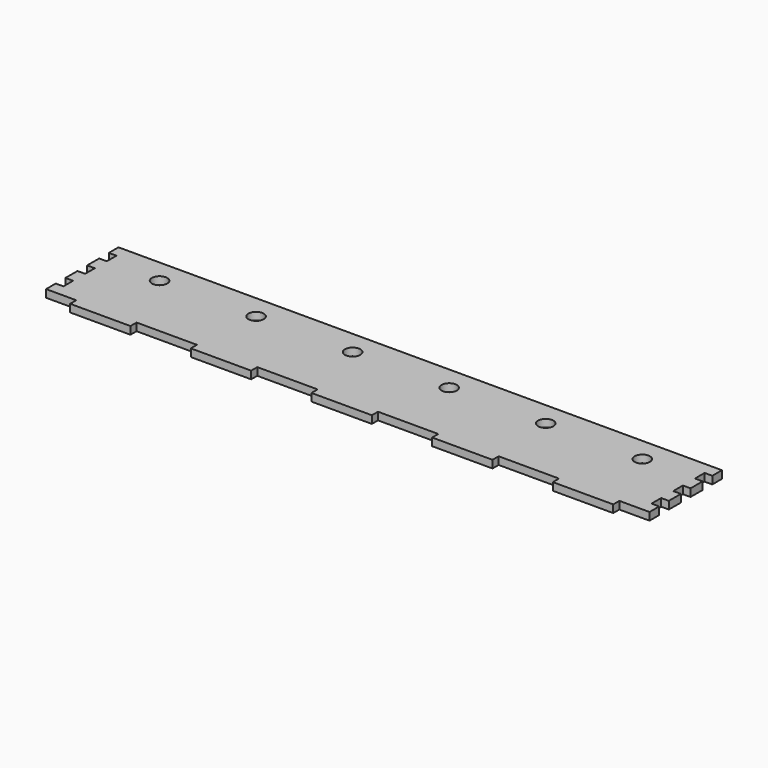
from build123d import *

# Parameters (mm, degrees)
F0_W     = 500
F0_H     = 75
F1_DEPTH = 6.35
F2_W     = 50
F2_H     = 6.35
F3_DEPTH = 6.35
F4_W     = 6.35
F4_H     = 10
F5_DEPTH = 6.351
F6_R     = 6.35
F7_DEPTH = 25


# Not quite as in the source:
# - a length typed as a fraction of an inch, garbled in the dataset ("3 / 203.2 mm" for 3/8 in), is restored


with BuildPart() as f1:
    # F0 (on Top) → F1 (new body)
    with BuildSketch(Plane.XY):
        Rectangle(F0_W, F0_H)
    extrude(amount=F1_DEPTH)

    # F2 (on face) → F3 (join, through all)
    with BuildSketch(Plane.XY.offset(6.35)):
        with Locations((-200, -40.675)):
            Rectangle(F2_W, F2_H)
        with Locations((-100, -40.675)):
            Rectangle(F2_W, F2_H)
        with Locations((0, -40.675)):
            Rectangle(F2_W, F2_H)
        with Locations((100, -40.675)):
            Rectangle(F2_W, F2_H)
        with Locations((200, -40.675)):
            Rectangle(F2_W, F2_H)
    extrude(amount=-F3_DEPTH)

    # F4 (on face) → F5 (cut, through all)
    with BuildSketch(Plane.XY.offset(6.35)):
        with Locations((246.825, 22.5)):
            Rectangle(F4_W, F4_H)
        with Locations((246.825, 0)):
            Rectangle(F4_W, F4_H)
        with Locations((246.825, -22.5)):
            Rectangle(F4_W, F4_H)
        with Locations((-246.825, 22.5)):
            Rectangle(F4_W, F4_H)
        with Locations((-246.825, 0)):
            Rectangle(F4_W, F4_H)
        with Locations((-246.825, -22.5)):
            Rectangle(F4_W, F4_H)
    extrude(amount=-F5_DEPTH, mode=Mode.SUBTRACT)

    # F6 (on face) → F7 (cut)
    with BuildSketch(Plane.XY.offset(6.35)):
        with Locations((-200, 17.5)):
            Circle(F6_R)
        with Locations((-120, 17.5)):
            Circle(F6_R)
        with Locations((-40, 17.5)):
            Circle(F6_R)
        with Locations((40, 17.5)):
            Circle(F6_R)
        with Locations((120, 17.5)):
            Circle(F6_R)
        with Locations((200, 17.5)):
            Circle(F6_R)
    extrude(amount=-F7_DEPTH, mode=Mode.SUBTRACT)


solid = f1.part
